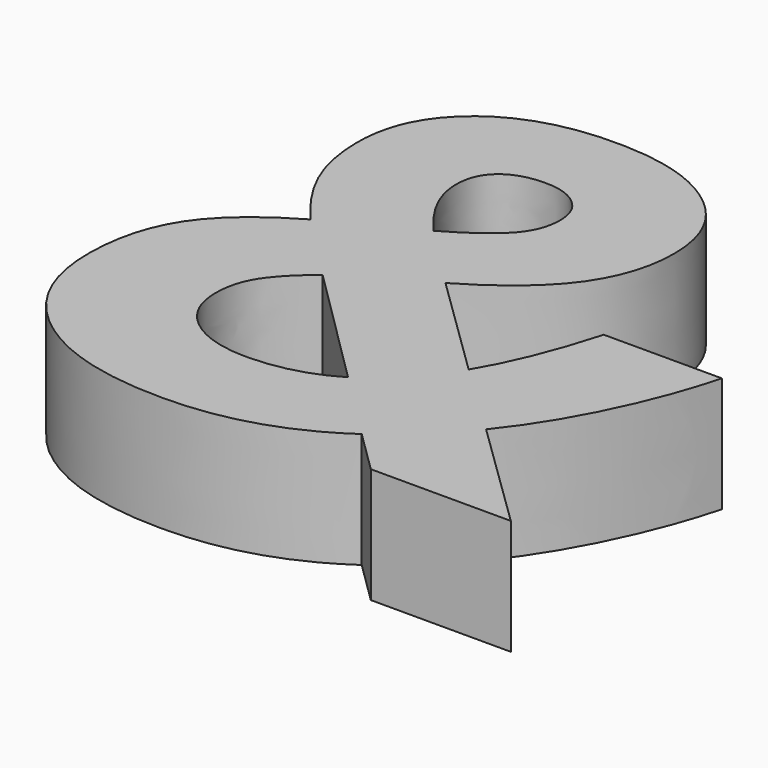
from build123d import *

# Parameters (mm, degrees)
F0_TEXT_SIZE = 66.0000032642
F1_DEPTH     = 10


# Not quite as in the source:
# - Text() gives the source's letters only with a copy of the font that has no kerning and outlines rounded to 1/6400 em; it was checked with that copy


with BuildPart() as f1:
    # F0 (on Top) → F1 (new body)
    with BuildSketch(Plane.XY):
        with Locations((-25.2899993211, -23.3100019395)):
            Text('&', F0_TEXT_SIZE, font='Open Sans', font_style=FontStyle.BOLD, text_align=(TextAlign.LEFT, TextAlign.BOTTOM))
    extrude(amount=F1_DEPTH)


solid = f1.part
